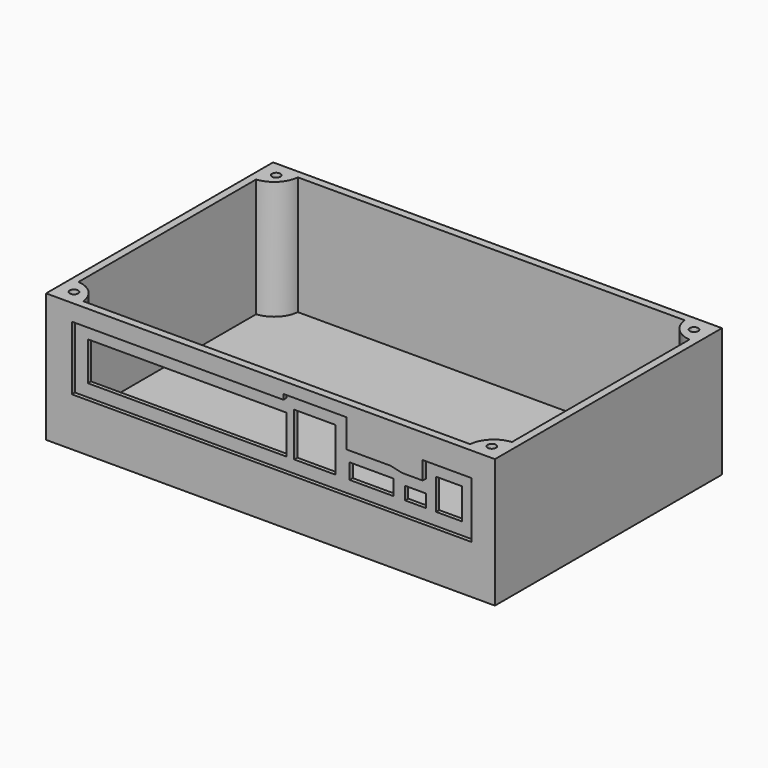
from build123d import *

# Parameters (mm, degrees)
F0_W         = 174
F0_H         = 110
F1_DEPTH     = 4
F2_W         = 174
F2_H         = 110
F2_W_2       = 168
F2_H_2       = 104
F3_DEPTH     = 46
F5_R         = 3.5
F6_DEPTH     = 2
F7_W         = 38.5
F7_H         = 15
F7_W_2       = 8
F7_H_2       = 17
F7_W_3       = 8.5
F7_H_3       = 6
F7_W_4       = 4
F7_H_4       = 5
F7_W_5       = 5
F7_H_5       = 12
F8_DEPTH     = 3
F9_W         = 9
F9_H         = 9
F9_R         = 1.63
F10_DEPTH    = 46
F11_DEPTH    = 50.001
F12_T1_DEPTH = 68.5
F13_R        = 3.63
F13_R_2      = 1.63
F14_DEPTH    = 2
F15_DEPTH    = 1.5


# Not quite as in the source:
# - a fillet or chamfer that OpenCascade refuses, or shapes differently, is made with other operations: its cross-section is extruded or revolved along the edge and cut away or added


with BuildPart() as f1:
    # F0 (on Top) → F1 (new body)
    with BuildSketch(Plane.XY):
        Rectangle(F0_W, F0_H)
    extrude(amount=-F1_DEPTH)

    # F2 (on face) → F3 (join)
    with BuildSketch(Plane.XY):
        Rectangle(F2_W, F2_H)
        Rectangle(F2_W_2, F2_H_2, mode=Mode.SUBTRACT)
    extrude(amount=F3_DEPTH)

    # F5 (on face) → F6 (cut)
    with BuildSketch(Plane(origin=(0, 0, -4), x_dir=(1, 0, 0), z_dir=(0, 0, -1))):
        with Locations((-66.7, 40.5)):
            Circle(F5_R)
        with Locations((-70, 26.5)):
            Circle(F5_R)
        with Locations((-66.7, -36.1)):
            Circle(F5_R)
        with Locations((-70, -46.5)):
            Circle(F5_R)
        with Locations((-5, -36.1)):
            Circle(F5_R)
        with Locations((5, -36.1)):
            Circle(F5_R)
        with Locations((-5, 40.5)):
            Circle(F5_R)
        with Locations((5, 40.5)):
            Circle(F5_R)
        with Locations((66.7, 40.5)):
            Circle(F5_R)
        with Locations((70, 26.5)):
            Circle(F5_R)
        with Locations((66.7, -36.1)):
            Circle(F5_R)
        with Locations((70, -46.5)):
            Circle(F5_R)
    extrude(amount=-F6_DEPTH, mode=Mode.SUBTRACT)

    # F7 (on face) → F8 (cut)
    with BuildSketch(Plane.XZ.offset(55)):
        with Locations((-52.75, 27.1)):
            Rectangle(F7_W, F7_H)
        with Locations((-14.25, 27.1)):
            Rectangle(F7_W, F7_H)
        with Locations((12, 28.1)):
            Rectangle(F7_W_2, F7_H_2)
        with Locations((20, 28.1)):
            Rectangle(F7_W_2, F7_H_2)
        with Locations((33.75, 22.6)):
            Rectangle(F7_W_3, F7_H_3)
        with Locations((42.25, 22.6)):
            Rectangle(F7_W_3, F7_H_3)
        with Locations((53, 22.1)):
            Rectangle(F7_W_4, F7_H_4)
        with Locations((57, 22.1)):
            Rectangle(F7_W_4, F7_H_4)
        with Locations((65.5, 25.6)):
            Rectangle(F7_W_5, F7_H_5)
        with Locations((70.5, 25.6)):
            Rectangle(F7_W_5, F7_H_5)
    extrude(amount=-F8_DEPTH, mode=Mode.SUBTRACT)

    # F9 (on face) → F10 (join)
    with BuildSketch(Plane.XY.offset(46)):
        with Locations((-79.5, 47.5)):
            Rectangle(F9_W, F9_H)
        with Locations((-81, 49)):
            Circle(F9_R, mode=Mode.SUBTRACT)
        Polygon((-75, 55), (-87, 55), (-87, 43), (-84, 43), (-84, 52), (-75, 52), align=None)
        Polygon((87, 55), (75, 55), (75, 52), (84, 52), (84, 43), (87, 43), align=None)
        with Locations((79.5, 47.5)):
            Rectangle(F9_W, F9_H)
        with Locations((81, 49)):
            Circle(F9_R, mode=Mode.SUBTRACT)
        Polygon((87, -55), (87, -43), (84, -43), (84, -52), (75, -52), (75, -55), align=None)
        with Locations((79.5, -47.5)):
            Rectangle(F9_W, F9_H)
        with Locations((81, -49)):
            Circle(F9_R, mode=Mode.SUBTRACT)
        with Locations((-79.5, -47.5)):
            Rectangle(F9_W, F9_H)
        with Locations((-81, -49)):
            Circle(F9_R, mode=Mode.SUBTRACT)
        Polygon((-84, -43), (-87, -43), (-87, -55), (-75, -55), (-75, -52), (-84, -52), align=None)
    extrude(amount=-F10_DEPTH)

    # F9 (on face) → F11 (cut, through all)
    with BuildSketch(Plane.XY.offset(46)):
        with Locations((-81, 49)):
            Circle(F9_R)
        with Locations((81, 49)):
            Circle(F9_R)
        with Locations((81, -49)):
            Circle(F9_R)
        with Locations((-81, -49)):
            Circle(F9_R)
    extrude(amount=-F11_DEPTH, mode=Mode.SUBTRACT)

    # F12: fillet of radius 10 on 4 edges, made by hand

    # F12_s2 → F12_t1 (cut)
    with BuildSketch(Plane.XY):
        with BuildLine():
            ThreePointArc((-75, 52), (-77.8832882455, 45.8832882455), (-84, 43))
            Line((-84, 43), (-75, 43))
            Line((-75, 43), (-75, 52))
        make_face()
        with BuildLine():
            ThreePointArc((84, 43), (77.8832882455, 45.8832882455), (75, 52))
            Line((75, 52), (75, 43))
            Line((75, 43), (84, 43))
        make_face()
        with BuildLine():
            ThreePointArc((-84, -43), (-77.8832882455, -45.8832882455), (-75, -52))
            Line((-75, -52), (-75, -43))
            Line((-75, -43), (-84, -43))
        make_face()
        with BuildLine():
            ThreePointArc((75, -52), (77.8832882455, -45.8832882455), (84, -43))
            Line((84, -43), (75, -43))
            Line((75, -43), (75, -52))
        make_face()
    extrude(amount=F12_T1_DEPTH, mode=Mode.SUBTRACT)

    # F13 (on face) → F14 (cut)
    with BuildSketch(Plane(origin=(0, 0, -4), x_dir=(1, 0, 0), z_dir=(0, 0, -1))):
        with Locations((-81, 49)):
            Circle(F13_R)
        with Locations((-81, 49)):
            Circle(F13_R_2, mode=Mode.SUBTRACT)
        with Locations((81, 49)):
            Circle(F13_R)
        with Locations((81, 49)):
            Circle(F13_R_2, mode=Mode.SUBTRACT)
        with Locations((81, -49)):
            Circle(F13_R)
        with Locations((81, -49)):
            Circle(F13_R_2, mode=Mode.SUBTRACT)
        with Locations((-81, -49)):
            Circle(F13_R)
        with Locations((-81, -49)):
            Circle(F13_R_2, mode=Mode.SUBTRACT)
    extrude(amount=-F14_DEPTH, mode=Mode.SUBTRACT)

    # F7 (on face) → F15 (cut)
    with BuildSketch(Plane.XZ.offset(55)):
        Polygon((-77, 34.6), (-77, 19.7916162387), (-77, 14.7916162387), (78, 14.7916162387), (78, 19.6), (78, 31.6), (78, 36.6), (73, 36.6), (68, 36.6), (63, 36.6), (59, 36.6), (59, 29.6), (55, 29.6), (51, 29.6), (46.5, 30.6), (38, 30.6), (29.5, 30.6), (29.5, 41.6), (24, 41.6), (16, 41.6), (8, 41.6), (5, 41.6), (5, 39.6), (-33.5, 39.6), (-72, 39.6), (-77, 39.6), align=None)
        Polygon((5, 19.6), (-33.5, 19.6), (-72, 19.6), (-72, 34.6), (-33.5, 34.6), (5, 34.6), align=None, mode=Mode.SUBTRACT)
        Polygon((46.5, 19.6), (38, 19.6), (29.5, 19.6), (29.5, 25.6), (38, 25.6), (46.5, 25.6), align=None, mode=Mode.SUBTRACT)
        Polygon((24, 19.6), (16, 19.6), (8, 19.6), (8, 36.6), (16, 36.6), (24, 36.6), align=None, mode=Mode.SUBTRACT)
        Polygon((59, 19.6), (55, 19.6), (51, 19.6), (51, 24.6), (55, 24.6), (59, 24.6), align=None, mode=Mode.SUBTRACT)
        Polygon((73, 19.6), (68, 19.6), (63, 19.6), (63, 31.6), (68, 31.6), (73, 31.6), align=None, mode=Mode.SUBTRACT)
    extrude(amount=-F15_DEPTH, mode=Mode.SUBTRACT)


solid = f1.part
